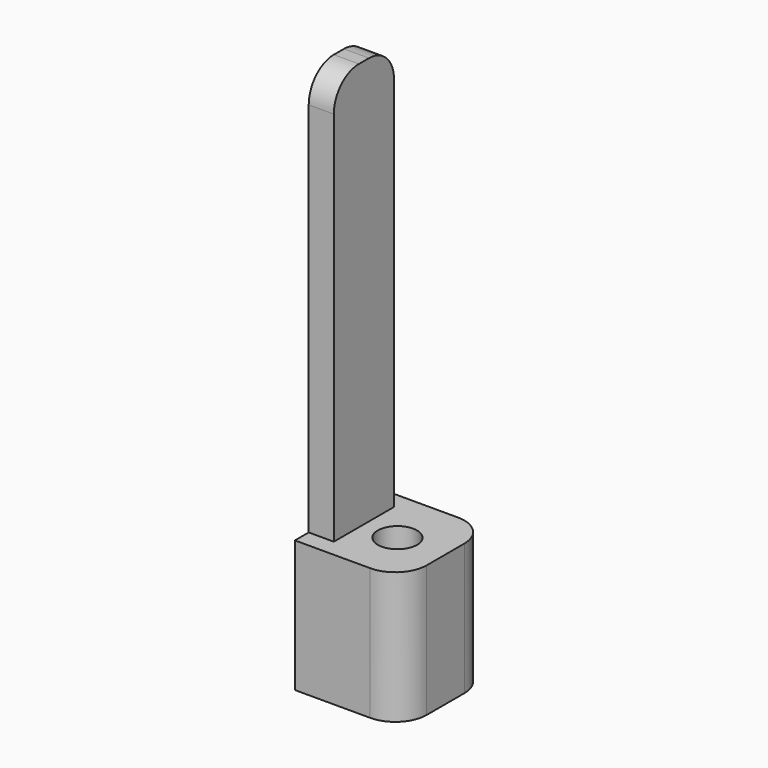
from build123d import *

# Parameters (mm, degrees)
F1_DEPTH  = 8.4
F2_R      = 2.5
F3_DEPTH  = 1.6
F4_R      = 1.25
F5_DEPTH  = 10
F6_W      = 2
F6_H      = 4.8
F7_DEPTH  = 26
F8_R      = 2
F9_DEPTH  = 0.2
F10_DEPTH = 0.2


# Not quite as in the source:
# - a feature names something its author has since deleted; it is built from what else it names


with BuildPart() as f1:
    # F0 (on Top) → F1 (new body)
    with BuildSketch(Plane.XY):
        with BuildLine():
            Line((1, 21.8148477226), (-4, 21.8148477226))
            Line((-4, 21.8148477226), (-4, 14.8148477226))
            Line((-4, 14.8148477226), (1, 14.8148477226))
            ThreePointArc((1, 14.8148477226), (2.4142135624, 15.4006341603), (3, 16.8148477226))
            Line((3, 16.8148477226), (3, 19.8148477226))
            ThreePointArc((3, 19.8148477226), (2.4142135624, 21.229061285), (1, 21.8148477226))
        make_face()
    extrude(amount=F1_DEPTH)

    # F2 (on face) → F3 (cut)
    with BuildSketch(Plane(origin=(0, 0, 0), x_dir=(1, 0, 0), z_dir=(0, 0, -1))):
        with Locations((0, -18.2346012443)):
            Circle(F2_R)
    extrude(amount=-F3_DEPTH, mode=Mode.SUBTRACT)

    # F4 (on face) → F5 (cut)
    with BuildSketch(Plane(origin=(0, 0, 1.6), x_dir=(1, 0, 0), z_dir=(0, 0, -1))):
        with Locations((0, -18.2346012443)):
            Circle(F4_R)
    extrude(amount=-F5_DEPTH, mode=Mode.SUBTRACT)

    # F6 (on face) → F7 (join)
    with BuildSketch(Plane.XY.offset(8.4)):
        with Locations((-3, 18.3148477226)):
            Rectangle(F6_W, F6_H)
    extrude(amount=F7_DEPTH)

    # F8
    f8_edges = [f1.edges().sort_by_distance(p)[0] for p in [
        (-3, 20.714848, 34.4),
        (-3, 15.914848, 34.4),
    ]]
    fillet(f8_edges, radius=F8_R)

    # F9 (cut): a face of the model
    f9_faces = [f1.faces().sort_by_distance(p)[0] for p in [
        (-2, 18.3148477226, 21.2249019293),
    ]]
    extrude(f9_faces, amount=-F9_DEPTH, mode=Mode.SUBTRACT)

    # F10 (cut): a face of the model
    f10_faces = [f1.faces().sort_by_distance(p)[0] for p in [
        (-4, 18.3148477226, 15.72101639),
    ]]
    extrude(f10_faces, amount=-F10_DEPTH, mode=Mode.SUBTRACT)


solid = f1.part
